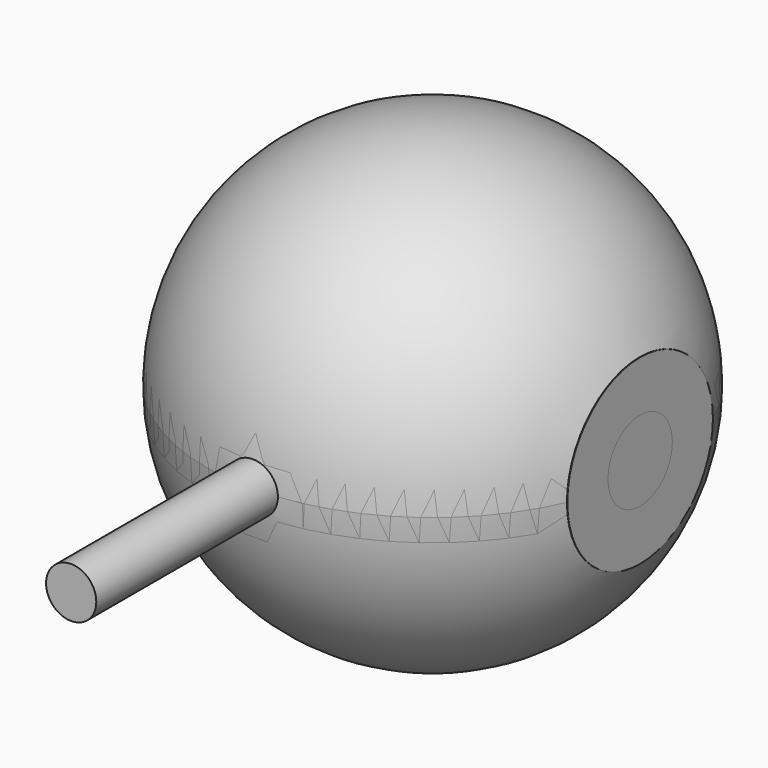
from build123d import *

# Parameters (mm, degrees)
F3_START  = 13.081
F2_R      = 5.7833610308
F3_DEPTH  = 1.2065
F4_R      = 2.54
F5_DEPTH  = 0.0254
F6_DEPTH  = 0.0254
F8_START  = -10.16
F7_R      = 0.762
F8_DEPTH  = 35.56
F9_R      = 1.5875
F10_DEPTH = 14.2875
F11_DEPTH = 28.5369


# Not quite as in the source:
# - a feature names something its author has since deleted; it is built from what else it names


with BuildPart() as f1:
    # F0 (on Front) → F1 (revolve)
    with BuildSketch(Plane.XZ):
        with BuildLine():
            ThreePointArc((0, -14.2875), (10.1027881362, -10.1027881362), (14.2875, 0))
            ThreePointArc((14.2875, 0), (10.1027881362, 10.1027881362), (0, 14.2875))
            Line((0, 14.2875), (0, -14.2875))
        make_face()
    revolve(axis=Axis((0, 0, 0), (0, 0, -1)))

    # F2 (on Right) → F3 (cut)
    with BuildSketch(Plane.YZ.offset(F3_START)):
        Circle(F2_R)
    extrude(amount=F3_DEPTH, mode=Mode.SUBTRACT)

    # F7 (on Top) → F8 (cut)
    with BuildSketch(Plane.XY.offset(F8_START)):
        Circle(F7_R)
    extrude(amount=-F8_DEPTH, mode=Mode.SUBTRACT)

    # F9 (on Front) → F10 (cut, through all)
    with BuildSketch(Plane.XZ):
        Circle(F9_R)
    extrude(amount=F10_DEPTH, mode=Mode.SUBTRACT)


with BuildPart() as f5:
    # F4 (on face) → F5 (new body)
    with BuildSketch(Plane.YZ.offset(13.081)):
        Circle(F4_R)
    extrude(amount=F5_DEPTH)


with BuildPart() as f6:
    # F4 (on face) → F6 (new body)
    with BuildSketch(Plane.YZ.offset(13.081)):
        with BuildLine():
            ThreePointArc((0, -5.7463114474), (4.0632557912, -4.0632557912), (5.7463114474, 0))
            ThreePointArc((5.7463114474, 0), (4.0632557912, 4.0632557912), (0, 5.7463114474))
            ThreePointArc((0, 5.7463114474), (-5.7463114474, 0), (0, -5.7463114474))
        make_face()
        Circle(F4_R, mode=Mode.SUBTRACT)
    extrude(amount=F6_DEPTH)


with BuildPart() as f11:
    # F11 (new): a face of the model
    f11_faces = [f1.part.faces().sort_by_distance(p)[0] for p in [
        (0, 0, 0),
    ]]
    extrude(f11_faces, amount=F11_DEPTH)


with BuildPart() as f12_1:
    # F12: instance of F1
    add(f1.part.mirror(Plane.XZ))


solid = Compound([f1.part, f5.part, f6.part, f11.part, f12_1.part])
